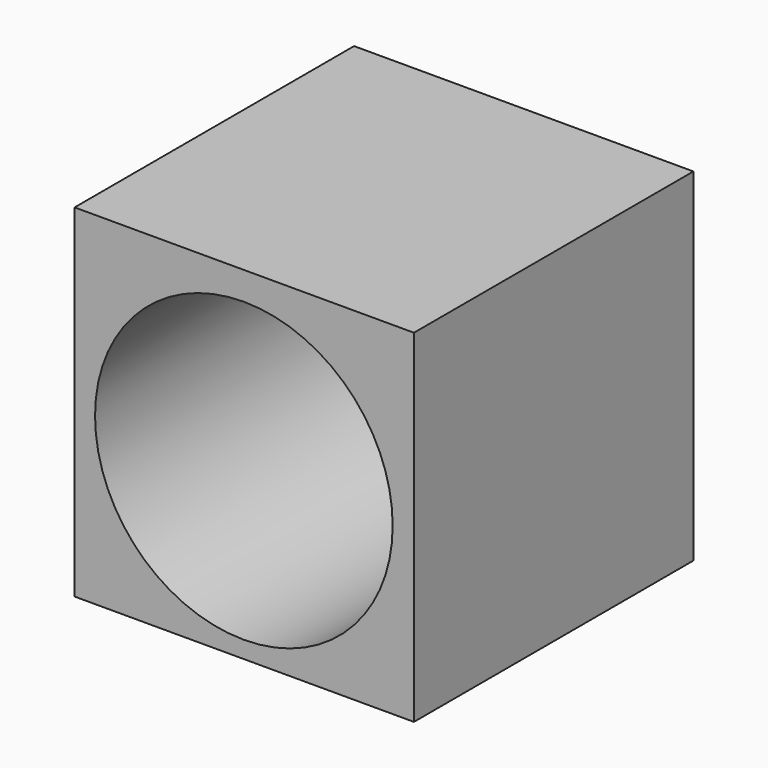
from build123d import *

# Parameters (mm, degrees)
F0_W     = 123.3636140823
F0_H     = 124.569028616
F0_R     = 54.1030855555
F1_DEPTH = 127


# Not quite as in the source:
# - the program builds the solid bodies; features that only make, move or delete a surface that nothing else refers to are left out


with BuildPart() as f1:
    # F0 (on Front) → F1 (new body)
    with BuildSketch(Plane.XZ):
        with Locations((0.1526474953, 2.0047873259)):
            Rectangle(F0_W, F0_H)
        Circle(F0_R, mode=Mode.SUBTRACT)
    extrude(amount=F1_DEPTH)


solid = f1.part
